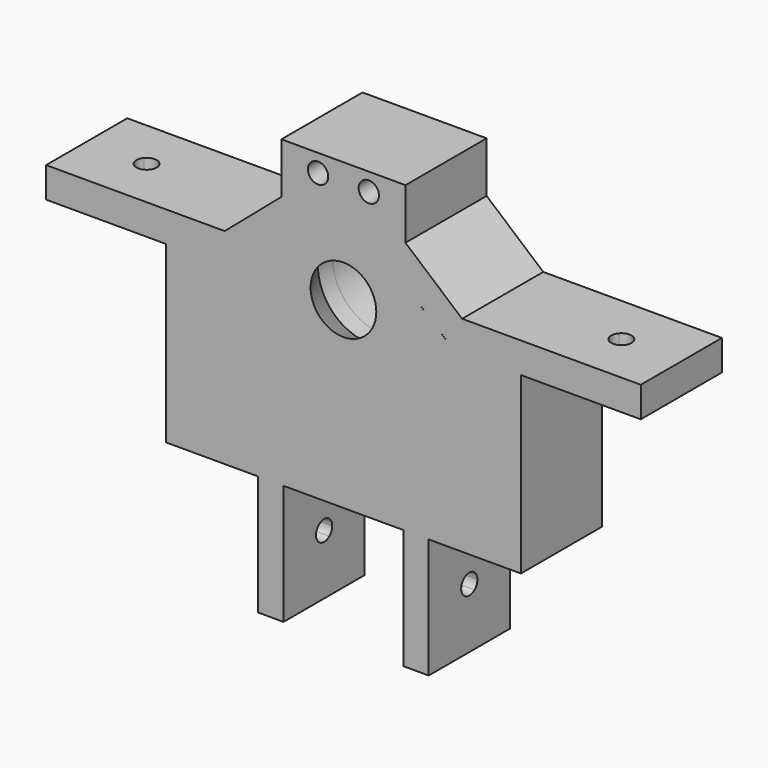
from build123d import *

# Parameters (mm, degrees)
F0_R        = 1.27
F0_R_2      = 3.96875
F1_DEPTH    = 6.35
F2_R        = 6.477
F2_R_2      = 1.27
F3_DEPTH    = 6.35
F4_S5_R     = 6.477
F4_T6_DEPTH = 13
F5_W        = 12.7
F5_H        = 3.81
F6_DEPTH    = 14.9999954
F8_DEPTH    = 25.4
F9_W        = 12.7
F9_H        = 3.81
F10_DEPTH   = 14.9999954
F12_DEPTH   = 25.4
F13_W       = 3.175
F13_H       = 12.7
F14_DEPTH   = 14.9999954
F16_DEPTH   = 25.4


# Not quite as in the source:
# - a fillet or chamfer that OpenCascade refuses, or shapes differently, is made with other operations: its cross-section is extruded or revolved along the edge and cut away or added
# - after a boolean that leaves OpenCascade's solid faulty, fix() repairs it
# - ends of sketch curves that miss each other by under 0.0002 mm in the source are joined


with BuildPart() as f1:
    # F0 (on Front) → F1 (new body)
    with BuildSketch(Plane.XZ):
        Polygon((-7.493, 0.1328983575), (0, 0.1328983575), (7.493, 0.1328983575), (22.2194990303, 0.1328983575), (22.2194990303, 19.5094533027), (14.8570176459, 25.8122983575), (7.7658264293, 31.8828983575), (7.7658264293, 38.2328983575), (-7.7713273633, 38.2328983575), (-7.7713273633, 31.8828983575), (-14.8625185798, 25.8122983575), (-22.2249999642, 19.5094533027), (-22.2249999642, 4.5234533027), (-22.2249999642, 0.1328983575), align=None)
        with Locations((-3.175, 36.0046029091)):
            Circle(F0_R, mode=Mode.SUBTRACT)
        with BuildLine():
            ThreePointArc((-1.6471995105, 13.7654938087), (-14.0416307026, 9.056743723), (-13.4701421127, 22.3031640975))
            Line((-13.4701421127, 22.3031640975), (-7.8430329322, 27.1203983575))
            Line((-7.8430329322, 27.1203983575), (-3.175, 27.1203983575))
            Line((-3.175, 27.1203983575), (-3.175, 30.2953983575))
            Line((-3.175, 30.2953983575), (-3.175, 33.4703983575))
            Line((-3.175, 33.4703983575), (3.175, 33.4703983575))
            Line((3.175, 33.4703983575), (3.175, 30.2953983575))
            Line((3.175, 30.2953983575), (3.175, 27.1203983575))
            Line((3.175, 27.1203983575), (7.8375319983, 27.1203983575))
            Line((7.8375319983, 27.1203983575), (13.4701421127, 22.3031640975))
            ThreePointArc((13.4701421127, 22.3031640975), (16.2995077669, 19.40684068), (17.3322006389, 15.4917998403))
            ThreePointArc((17.3322006389, 15.4917998403), (10.2711150187, 7.6028326022), (1.6507381924, 13.7496885133))
            ThreePointArc((1.6507381924, 13.7496885133), (0.0063534061, 14.7141035739), (-1.6471995105, 13.7654938087))
        make_face(mode=Mode.SUBTRACT)
        with Locations((3.175, 36.0046029091)):
            Circle(F0_R, mode=Mode.SUBTRACT)
        Polygon((14.8570176459, 25.8122983575), (22.2194990303, 19.5094533027), (22.2194990303, 25.8122983575), (17.4187807526, 25.8122983575), align=None)
        Polygon((-22.2249999642, 25.8122983575), (-22.2249999642, 19.5094533027), (-14.8625185798, 25.8122983575), (-17.4242816865, 25.8122983575), align=None)
        with BuildLine():
            ThreePointArc((13.4519986436, 22.3139871107), (4.7326542757, 21.9159130054), (1.6507381924, 13.7496885133))
            ThreePointArc((1.6507381924, 13.7496885133), (10.2711150187, 7.6028326022), (17.3322006389, 15.4917998403))
            ThreePointArc((17.3322006389, 15.4917998403), (16.2995077669, 19.40684068), (13.4701421127, 22.3031640975))
            ThreePointArc((13.4701421127, 22.3031640975), (13.461073979, 22.3085816404), (13.4519986436, 22.3139871107))
        make_face()
        with BuildLine():
            ThreePointArc((-1.4572006389, 15.4917998403), (-5.4796598384, 22.3966069904), (-13.4701421898, 22.3031640514))
            ThreePointArc((-13.4701421127, 22.3031640975), (-14.0416307026, 9.056743723), (-1.6471995105, 13.7654938087))
            ThreePointArc((-1.6471995105, 13.7654938087), (-1.5048433381, 14.6234346974), (-1.4572006389, 15.4917998403))
        make_face()
        with BuildLine():
            Line((-7.8430329322, 27.1203983575), (-13.4701422669, 22.3031640053))
            ThreePointArc((-13.4701421898, 22.3031640514), (-5.4796598384, 22.3966069904), (-1.4572006389, 15.4917998403))
            ThreePointArc((-1.4572006389, 15.4917998403), (-1.5048433381, 14.6234346974), (-1.6471995105, 13.7654938087))
            ThreePointArc((-1.6471995105, 13.7654938087), (0.0063534061, 14.7141035739), (1.6507381924, 13.7496885133))
            ThreePointArc((1.6507381924, 13.7496885133), (4.7326542757, 21.9159130054), (13.4519986436, 22.3139871107))
            Line((13.4519986436, 22.3139871107), (7.8375319983, 27.1203983575))
            Line((7.8375319983, 27.1203983575), (3.175, 27.1203983575))
            Line((3.175, 27.1203983575), (3.175, 30.2953983575))
            Line((3.175, 30.2953983575), (3.175, 33.4703983575))
            Line((3.175, 33.4703983575), (-3.175, 33.4703983575))
            Line((-3.175, 33.4703983575), (-3.175, 30.2953983575))
            Line((-3.175, 30.2953983575), (-3.175, 27.1203983575))
            Line((-3.175, 27.1203983575), (-7.8430329322, 27.1203983575))
        make_face()
        with Locations((0, 23.0759866536)):
            Circle(F0_R_2, mode=Mode.SUBTRACT)
    extrude(amount=F1_DEPTH)

    # F2 (on face) → F3 (join)
    with BuildSketch(Plane(origin=(0, 0, 0), x_dir=(-1, 0, 0), z_dir=(0, 1, 0))):
        Polygon((-22.2194990303, 25.8122983575), (-22.2194990303, 0.1328983575), (22.2249999642, 0.1328983575), (22.2249999642, 25.8122983575), (14.8625185798, 25.8122983575), (7.7713273633, 31.8828983575), (7.7713273633, 38.2328983575), (-7.7658264293, 38.2328983575), (-7.7658264293, 31.8828983575), (-14.8570176459, 25.8122983575), align=None)
        with Locations((0, 23.0759866536)):
            Circle(F2_R, mode=Mode.SUBTRACT)
        with Locations((-3.175, 36.0046029091)):
            Circle(F2_R_2, mode=Mode.SUBTRACT)
        with Locations((3.175, 36.0046029091)):
            Circle(F2_R_2, mode=Mode.SUBTRACT)
    extrude(amount=F3_DEPTH)

    # F4: chamfer of 3.81 x 6.5991135768 on 1 edges, made by hand


with BuildPart() as f4_tool2:
    # F4_s3 → F4_t4 (revolve)
    with BuildSketch(Plane.XY.offset(23.0759866536)):
        Polygon((7.77875, 0), (3.96875, -6.5991135768), (3.96875, 0), align=None)
    revolve(axis=Axis((0, 0, 23.0759866536), (0, -1, 0)))

    # F4_s5 → F4_t6 (intersect, symmetric)
    with BuildSketch(Plane.XZ.offset(3.3)):
        with Locations((0, 23.0759866536)):
            Circle(F4_S5_R)
    extrude(amount=F4_T6_DEPTH, both=True, mode=Mode.INTERSECT)


with BuildPart() as f1_1:
    add(f1.part)

    # F4_t1: cut F4_tool2
    add(f4_tool2.part, mode=Mode.SUBTRACT)

    # F5 (on face) → F6 (join)
    with BuildSketch(Plane(origin=(-22.2249999642, 0, 0), x_dir=(0, -1, 0), z_dir=(-1, 0, 0))):
        with Locations((0, 23.9072983575)):
            Rectangle(F5_W, F5_H)
    extrude(amount=F6_DEPTH)

    # F7 (on face) → F8 (cut)
    with BuildSketch(Plane(origin=(0, 0, 22.0022983575), x_dir=(1, 0, 0), z_dir=(0, 0, -1))):
        with BuildLine():
            ThreePointArc((-28.7557423483, 0.8206364192), (-30.5456340834, 0.969255316), (-30.6942529802, -0.8206364192))
            Line((-30.6942529802, -0.8206364192), (-28.7557423483, 0.8206364192))
        make_face()
        with BuildLine():
            Line((-28.7557423483, 0.8206364192), (-30.6942529802, -0.8206364192))
            ThreePointArc((-30.6942529802, -0.8206364192), (-29.2879932313, -1.1924458586), (-28.4549976642, 0))
            ThreePointArc((-28.4549976642, 0), (-28.5325518057, 0.4370044329), (-28.7557423483, 0.8206364192))
        make_face()
    extrude(amount=-F8_DEPTH, mode=Mode.SUBTRACT)

    # F9 (on face) → F10 (join)
    with BuildSketch(Plane.YZ.offset(22.2194990303)):
        with Locations((0, 23.9072983575)):
            Rectangle(F9_W, F9_H)
    extrude(amount=F10_DEPTH)

    # F11 (on face) → F12 (cut)
    with BuildSketch(Plane(origin=(0, 0, 22.0022983575), x_dir=(1, 0, 0), z_dir=(0, 0, -1))):
        with BuildLine():
            ThreePointArc((30.9894967303, 0), (30.9119425889, 0.4370044329), (30.6887520463, 0.8206364192))
            Line((30.6887520463, 0.8206364192), (28.7502414143, -0.8206364192))
            ThreePointArc((28.7502414143, -0.8206364192), (30.1565011632, -1.1924458586), (30.9894967303, 0))
        make_face()
        with BuildLine():
            Line((28.7502414143, -0.8206364192), (30.6887520463, 0.8206364192))
            ThreePointArc((30.6887520463, 0.8206364192), (28.8988603111, 0.969255316), (28.7502414143, -0.8206364192))
        make_face()
    extrude(amount=-F12_DEPTH, mode=Mode.SUBTRACT)

    # F13 (on face) → F14 (join)
    with BuildSketch(Plane(origin=(0, 0, 0.1328983575), x_dir=(1, 0, 0), z_dir=(0, 0, -1))):
        with Locations((9.0874977, 0)):
            Rectangle(F13_W, F13_H)
        with Locations((-9.0874977, 0)):
            Rectangle(F13_W, F13_H)
    extrude(amount=F14_DEPTH)

    add(f1_1.part.fix(), mode=Mode.REPLACE)

    # F15 (on face) → F16 (cut)
    with BuildSketch(Plane.YZ.offset(10.6749977)):
        with BuildLine():
            ThreePointArc((1.27, -7.3670993425), (0.5341777549, -6.2149039918), (-0.8206364192, -6.3978440265))
            Line((-0.8206364192, -6.3978440265), (0.8206364192, -8.3363546585))
            ThreePointArc((0.8206364192, -8.3363546585), (1.1521953507, -7.9012770974), (1.27, -7.3670993425))
        make_face()
        with BuildLine():
            Line((0.8206364192, -8.3363546585), (-0.8206364192, -6.3978440265))
            ThreePointArc((-0.8206364192, -6.3978440265), (-0.969255316, -8.1877357617), (0.8206364192, -8.3363546585))
        make_face()
    extrude(amount=-F16_DEPTH, mode=Mode.SUBTRACT)


solid = f1_1.part
